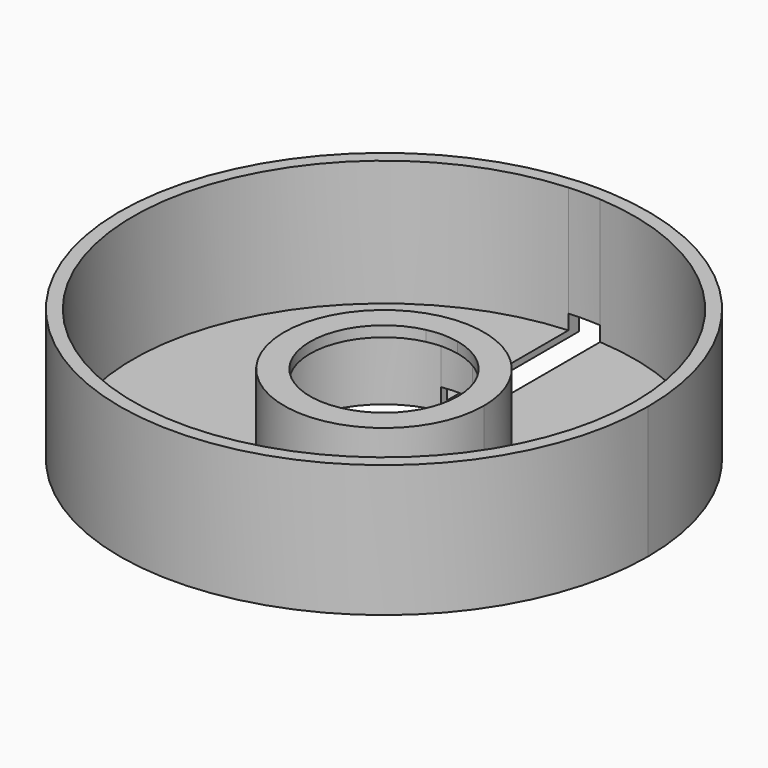
from build123d import *

# Parameters (mm, degrees)
F1_DEPTH = 15
F2_DEPTH = 13
F3_DEPTH = 1.2
F4_DEPTH = 25
F5_DEPTH = 4


with BuildPart() as f1:
    # F0 (on Top) → F1 (new body)
    with BuildSketch(Plane.XY):
        with BuildLine():
            ThreePointArc((-3, 17.2409396496), (0, 17.5), (3, 17.2409396496))
            Line((3, 17.2409396496), (3, 18.6603858481))
            ThreePointArc((3, 18.6603858481), (0, 18.9), (-3, 18.6603858481))
            Line((-3, 18.6603858481), (-3, 17.2409396496))
        make_face()
        with BuildLine():
            Line((3, 18.6603858481), (3, 17.2409396496))
            ThreePointArc((3, 17.2409396496), (13.393095236, 11.2638803261), (17.5, 0))
            ThreePointArc((17.5, 0), (-11.2638803261, -13.393095236), (-3, 17.2409396496))
            Line((-3, 17.2409396496), (-3, 18.6603858481))
            ThreePointArc((-3, 18.6603858481), (-12.2578546247, -14.3859306268), (18.9, 0))
            ThreePointArc((18.9, 0), (14.3859306268, 12.2578546247), (3, 18.6603858481))
        make_face()
        with BuildLine():
            ThreePointArc((-3, 13.6747943312), (0, 14), (3, 13.6747943312))
            Line((3, 13.6747943312), (3, 17.2409396496))
            ThreePointArc((3, 17.2409396496), (0, 17.5), (-3, 17.2409396496))
            Line((-3, 17.2409396496), (-3, 13.6747943312))
        make_face()
        with BuildLine():
            ThreePointArc((3, 13.6747943312), (10.9087121146, 8.7749643874), (14, 0))
            ThreePointArc((14, 0), (-8.7749643874, -10.9087121146), (-3, 13.6747943312))
            Line((-3, 13.6747943312), (-3, 17.2409396496))
            ThreePointArc((-3, 17.2409396496), (-11.2638803261, -13.393095236), (17.5, 0))
            ThreePointArc((17.5, 0), (13.393095236, 11.2638803261), (3, 17.2409396496))
            Line((3, 17.2409396496), (3, 13.6747943312))
        make_face()
    extrude(amount=F1_DEPTH)

    # F0 (on Top) → F2 (cut)
    with BuildSketch(Plane.XY):
        with BuildLine():
            ThreePointArc((-3, 13.6747943312), (0, 14), (3, 13.6747943312))
            Line((3, 13.6747943312), (3, 17.2409396496))
            ThreePointArc((3, 17.2409396496), (0, 17.5), (-3, 17.2409396496))
            Line((-3, 17.2409396496), (-3, 13.6747943312))
        make_face()
        with BuildLine():
            ThreePointArc((3, 13.6747943312), (10.9087121146, 8.7749643874), (14, 0))
            ThreePointArc((14, 0), (-8.7749643874, -10.9087121146), (-3, 13.6747943312))
            Line((-3, 13.6747943312), (-3, 17.2409396496))
            ThreePointArc((-3, 17.2409396496), (-11.2638803261, -13.393095236), (17.5, 0))
            ThreePointArc((17.5, 0), (13.393095236, 11.2638803261), (3, 17.2409396496))
            Line((3, 17.2409396496), (3, 13.6747943312))
        make_face()
    extrude(amount=F2_DEPTH, mode=Mode.SUBTRACT)

    # F0 (on Top) → F3 (join)
    with BuildSketch(Plane.XY):
        with BuildLine():
            ThreePointArc((-3, 18.6603858481), (0, 18.9), (3, 18.6603858481))
            Line((3, 18.6603858481), (3, 47.4051684946))
            ThreePointArc((3, 47.4051684946), (0, 47.5), (-3, 47.4051684946))
            Line((-3, 47.4051684946), (-3, 18.6603858481))
        make_face()
        with BuildLine():
            Line((3, 47.4051684946), (3, 18.6603858481))
            ThreePointArc((3, 18.6603858481), (14.3859306268, 12.2578546247), (18.9, 0))
            ThreePointArc((18.9, 0), (-12.2578546247, -14.3859306268), (-3, 18.6603858481))
            Line((-3, 18.6603858481), (-3, 47.4051684946))
            ThreePointArc((-3, 47.4051684946), (-32.5096139626, -34.6319938785), (47.5, 0))
            ThreePointArc((47.5, 0), (34.6319938785, 32.5096139626), (3, 47.4051684946))
        make_face()
    extrude(amount=F3_DEPTH)

    # F0 (on Top) → F4 (join)
    with BuildSketch(Plane.XY):
        with BuildLine():
            ThreePointArc((-3, 47.4051684946), (0, 47.5), (3, 47.4051684946))
            Line((3, 47.4051684946), (3, 49.9099188539))
            ThreePointArc((3, 49.9099188539), (0, 50), (-3, 49.9099188539))
            Line((-3, 49.9099188539), (-3, 47.4051684946))
        make_face()
        with BuildLine():
            Line((3, 49.9099188539), (3, 47.4051684946))
            ThreePointArc((3, 47.4051684946), (34.6319938785, 32.5096139626), (47.5, 0))
            ThreePointArc((47.5, 0), (-32.5096139626, -34.6319938785), (-3, 47.4051684946))
            Line((-3, 47.4051684946), (-3, 49.9099188539))
            ThreePointArc((-3, 49.9099188539), (-34.278273002, -36.4005494464), (50, 0))
            ThreePointArc((50, 0), (36.4005494464, 34.278273002), (3, 49.9099188539))
        make_face()
    extrude(amount=F4_DEPTH)

    # F0 (on Top) → F5 (cut)
    with BuildSketch(Plane.XY):
        with BuildLine():
            ThreePointArc((-3, 17.2409396496), (0, 17.5), (3, 17.2409396496))
            Line((3, 17.2409396496), (3, 18.6603858481))
            ThreePointArc((3, 18.6603858481), (0, 18.9), (-3, 18.6603858481))
            Line((-3, 18.6603858481), (-3, 17.2409396496))
        make_face()
        with BuildLine():
            ThreePointArc((-3, 18.6603858481), (0, 18.9), (3, 18.6603858481))
            Line((3, 18.6603858481), (3, 47.4051684946))
            ThreePointArc((3, 47.4051684946), (0, 47.5), (-3, 47.4051684946))
            Line((-3, 47.4051684946), (-3, 18.6603858481))
        make_face()
        with BuildLine():
            ThreePointArc((-3, 47.4051684946), (0, 47.5), (3, 47.4051684946))
            Line((3, 47.4051684946), (3, 49.9099188539))
            ThreePointArc((3, 49.9099188539), (0, 50), (-3, 49.9099188539))
            Line((-3, 49.9099188539), (-3, 47.4051684946))
        make_face()
    extrude(amount=F5_DEPTH, mode=Mode.SUBTRACT)


solid = f1.part
